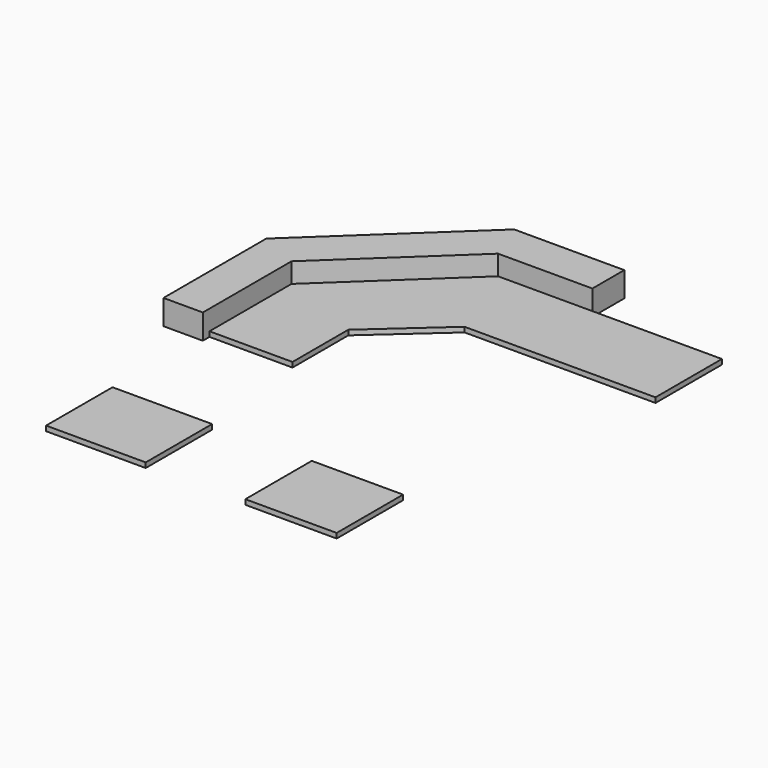
from build123d import *

# Parameters (mm, degrees)
F1_DEPTH = 38.1
F2_DEPTH = 190.5
F3_W     = 762
F3_H     = 635
F4_DEPTH = 38.1
F3_W_2   = 698.5


# Not quite as in the source:
# - a feature names something its author has since deleted; it is built from what else it names


with BuildPart() as f1:
    # F0 (on Top) → F1 (new body)
    with BuildSketch(Plane.XY):
        Polygon((-1460.5, 0), (0, 0), (0, 635), (-990.6, 635), (-1712.1399633702, 635), (-2613.764655485, -212.725), (-2613.764655485, -996.95), (-1978.764655485, -996.95), (-1978.764655485, -463.55), align=None)
    extrude(amount=F1_DEPTH)

    # F0 (on Top) → F2 (join)
    with BuildSketch(Plane.XY):
        Polygon((-1712.1399633702, 635), (-990.6, 635), (-990.6, 939.8), (-1832.9271457878, 939.8), (-2914.8946478161, -77.4868031215), (-2914.8946478161, -1060.45), (-2613.764655485, -1060.45), (-2613.764655485, -996.95), (-2613.764655485, -212.725), align=None)
    extrude(amount=F2_DEPTH)


with BuildPart() as f4:
    # F3 (on Top) → F4 (new body)
    with BuildSketch(Plane.XY):
        with Locations((-2232.764655485, -2241.55)):
            Rectangle(F3_W, F3_H)
    extrude(amount=F4_DEPTH)


with BuildPart() as f4b:
    # F3 (on Top) → F4, piece 2 (new body)
    with BuildSketch(Plane.XY):
        with Locations((-740.514655485, -2241.55)):
            Rectangle(F3_W_2, F3_H)
    extrude(amount=F4_DEPTH)


solid = Compound([f1.part, f4.part, f4b.part])
